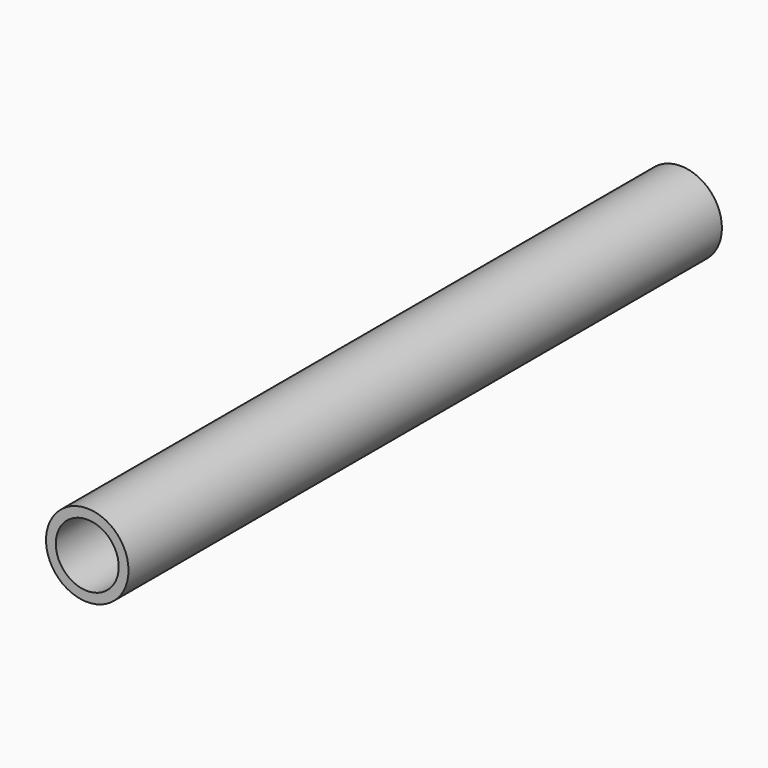
from build123d import *

# Parameters (mm, degrees)
F0_R          = 6.9211089712
F0_R_2        = 5.2800956232
F1_DEPTH      = 62.23
F1_DEPTH_BACK = 62.23
F4_DEPTH      = 25.4


# Not quite as in the source:
# - the program builds the solid bodies; features that only make, move or delete a surface that nothing else refers to are left out


with BuildPart() as f1:
    # F0 (on Front) → F1 (new body, two sides)
    with BuildSketch(Plane.XZ) as f1_sk:
        Circle(F0_R)
        Circle(F0_R_2, mode=Mode.SUBTRACT)
    extrude(amount=F1_DEPTH)
    extrude(f1_sk.sketch, amount=-F1_DEPTH_BACK)

    # F0 (on Front) → F4 (join)
    with BuildSketch(Plane.XZ):
        Circle(F0_R)
        Circle(F0_R_2, mode=Mode.SUBTRACT)
    extrude(amount=F4_DEPTH)


solid = f1.part
